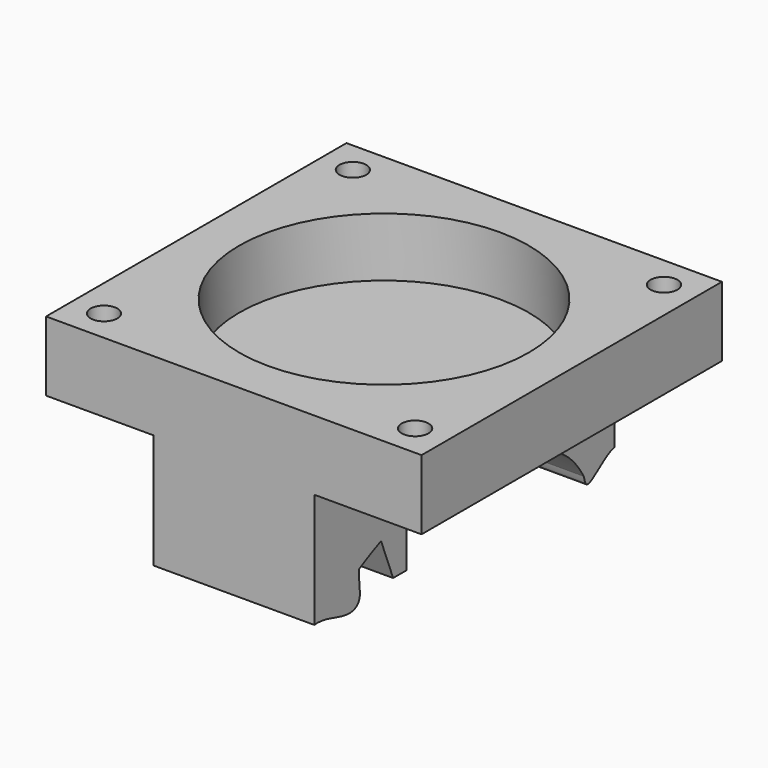
from build123d import *

# Parameters (mm, degrees)
F0_W       = 35
F0_H       = 35
F0_W_2     = 23
F0_H_2     = 23
F1_DEPTH   = 2
F3_DEPTH   = 5.5
F4_DEPTH   = 2.5
F5_DEPTH   = 1
F7_W       = 35
F7_H       = 35
F7_R       = 13.5
F8_DEPTH   = 1
F9_D       = 2.5
F9_DEPTH   = 10
F9_TIP     = 0.7510757738
F9_2_D     = 2.5
F9_2_DEPTH = 10
F9_2_TIP   = 0.7510757738
F10_W      = 7.5
F10_H      = 17.5
F11_DEPTH  = 25
F14_DEPTH  = 25


with BuildPart() as f1:
    # F0 (on Top) → F1 (new body)
    with BuildSketch(Plane.XY):
        with Locations((-9.5, 9.5)):
            Rectangle(F0_W, F0_H)
        with Locations((-9.5, 9.5)):
            Rectangle(F0_W_2, F0_H_2, mode=Mode.SUBTRACT)
        with Locations((-9.5, 9.5)):
            Rectangle(F0_W_2, F0_H_2)
        with BuildLine():
            Line((0, 5.027864045), (0, 0))
            Line((0, 0), (-5.027864045, 0))
            ThreePointArc((-5.027864045, 0), (-9.5, -1), (-13.972135955, 0))
            Line((-13.972135955, 0), (-19, 0))
            Line((-19, 0), (-19, 5.027864045))
            ThreePointArc((-19, 5.027864045), (-20, 9.5), (-19, 13.972135955))
            Line((-19, 13.972135955), (-19, 19))
            Line((-19, 19), (-13.972135955, 19))
            ThreePointArc((-13.972135955, 19), (-9.5, 20), (-5.027864045, 19))
            Line((-5.027864045, 19), (0, 19))
            Line((0, 19), (0, 13.972135955))
            ThreePointArc((0, 13.972135955), (0.746950766, 11.7912878475), (1, 9.5))
            ThreePointArc((1, 9.5), (0.746950766, 7.2087121525), (0, 5.027864045))
        make_face(mode=Mode.SUBTRACT)
        with BuildLine():
            Line((-13.972135955, 0), (-5.027864045, 0))
            ThreePointArc((-5.027864045, 0), (-2.0753787975, 2.0753787975), (0, 5.027864045))
            Line((0, 5.027864045), (0, 13.972135955))
            ThreePointArc((0, 13.972135955), (-2.0753787975, 16.9246212025), (-5.027864045, 19))
            Line((-5.027864045, 19), (-13.972135955, 19))
            ThreePointArc((-13.972135955, 19), (-16.9246212025, 16.9246212025), (-19, 13.972135955))
            Line((-19, 13.972135955), (-19, 5.027864045))
            ThreePointArc((-19, 5.027864045), (-16.9246212025, 2.0753787975), (-13.972135955, 0))
        make_face()
        with BuildLine():
            Line((-19, 19), (-19, 13.972135955))
            ThreePointArc((-19, 13.972135955), (-16.9246212025, 16.9246212025), (-13.972135955, 19))
            Line((-13.972135955, 19), (-19, 19))
        make_face()
        with BuildLine():
            ThreePointArc((-5.027864045, 19), (-2.0753787975, 16.9246212025), (0, 13.972135955))
            Line((0, 13.972135955), (0, 19))
            Line((0, 19), (-5.027864045, 19))
        make_face()
        with BuildLine():
            Line((-5.027864045, 0), (0, 0))
            Line((0, 0), (0, 5.027864045))
            ThreePointArc((0, 5.027864045), (-2.0753787975, 2.0753787975), (-5.027864045, 0))
        make_face()
        with BuildLine():
            Line((-19, 0), (-13.972135955, 0))
            ThreePointArc((-13.972135955, 0), (-16.9246212025, 2.0753787975), (-19, 5.027864045))
            Line((-19, 5.027864045), (-19, 0))
        make_face()
        with BuildLine():
            Line((0, 13.972135955), (0, 5.027864045))
            ThreePointArc((0, 5.027864045), (0.746950766, 7.2087121525), (1, 9.5))
            ThreePointArc((1, 9.5), (0.746950766, 11.7912878475), (0, 13.972135955))
        make_face()
        with BuildLine():
            ThreePointArc((-13.972135955, 0), (-9.5, -1), (-5.027864045, 0))
            Line((-5.027864045, 0), (-13.972135955, 0))
        make_face()
        with BuildLine():
            ThreePointArc((-19, 13.972135955), (-20, 9.5), (-19, 5.027864045))
            Line((-19, 5.027864045), (-19, 13.972135955))
        make_face()
        with BuildLine():
            Line((-13.972135955, 19), (-5.027864045, 19))
            ThreePointArc((-5.027864045, 19), (-9.5, 20), (-13.972135955, 19))
        make_face()
    extrude(amount=-F1_DEPTH)

    # F0 (on Top) → F4 (join)
    with BuildSketch(Plane.XY):
        with Locations((-9.5, 9.5)):
            Rectangle(F0_W_2, F0_H_2)
        with BuildLine():
            Line((0, 5.027864045), (0, 0))
            Line((0, 0), (-5.027864045, 0))
            ThreePointArc((-5.027864045, 0), (-9.5, -1), (-13.972135955, 0))
            Line((-13.972135955, 0), (-19, 0))
            Line((-19, 0), (-19, 5.027864045))
            ThreePointArc((-19, 5.027864045), (-20, 9.5), (-19, 13.972135955))
            Line((-19, 13.972135955), (-19, 19))
            Line((-19, 19), (-13.972135955, 19))
            ThreePointArc((-13.972135955, 19), (-9.5, 20), (-5.027864045, 19))
            Line((-5.027864045, 19), (0, 19))
            Line((0, 19), (0, 13.972135955))
            ThreePointArc((0, 13.972135955), (0.746950766, 11.7912878475), (1, 9.5))
            ThreePointArc((1, 9.5), (0.746950766, 7.2087121525), (0, 5.027864045))
        make_face(mode=Mode.SUBTRACT)
        with BuildLine():
            ThreePointArc((-19, 13.972135955), (-20, 9.5), (-19, 5.027864045))
            Line((-19, 5.027864045), (-19, 13.972135955))
        make_face()
        with BuildLine():
            Line((-13.972135955, 19), (-5.027864045, 19))
            ThreePointArc((-5.027864045, 19), (-9.5, 20), (-13.972135955, 19))
        make_face()
        with BuildLine():
            Line((0, 13.972135955), (0, 5.027864045))
            ThreePointArc((0, 5.027864045), (0.746950766, 7.2087121525), (1, 9.5))
            ThreePointArc((1, 9.5), (0.746950766, 11.7912878475), (0, 13.972135955))
        make_face()
        with BuildLine():
            ThreePointArc((-13.972135955, 0), (-9.5, -1), (-5.027864045, 0))
            Line((-5.027864045, 0), (-13.972135955, 0))
        make_face()
    extrude(amount=F4_DEPTH)


with BuildPart() as f3:
    # F2 (on face) → F3 (new body)
    with BuildSketch(Plane(origin=(0, 0, -2), x_dir=(1, 0, 0), z_dir=(0, 0, -1))):
        with BuildLine():
            Line((-27, -9.5), (-27, -27))
            Line((-27, -27), (8, -27))
            Line((8, -27), (8, -9.5))
            Line((8, -9.5), (4, -9.5))
            ThreePointArc((4, -9.5), (-9.5, -23), (-23, -9.5))
            Line((-23, -9.5), (-27, -9.5))
        make_face()
        with BuildLine():
            Line((-27, 8), (-27, -9.5))
            Line((-27, -9.5), (-23, -9.5))
            ThreePointArc((-23, -9.5), (-9.5, 4), (4, -9.5))
            Line((4, -9.5), (8, -9.5))
            Line((8, -9.5), (8, 8))
            Line((8, 8), (-27, 8))
        make_face()
    extrude(amount=F3_DEPTH)


with BuildPart() as f5:
    # F5 (new): a face of the model
    f5_faces = [f3.part.faces().sort_by_distance(p)[0] for p in [
        (-9.5, 26.5050252532, -7.5),
    ]]
    extrude(f5_faces, amount=F5_DEPTH)


with BuildPart() as f5b:
    # F5#2 (new): a face of the model
    f5_2_faces = [f1.part.faces().sort_by_distance(p)[0] for p in [
        (-9.5, 9.5, -2),
    ]]
    extrude(f5_2_faces, amount=F5_DEPTH)


with BuildPart() as f3_1:
    add(f3.part)

    # F7 (on face) → F8 (join)
    with BuildSketch(Plane(origin=(0, 0, -7.5), x_dir=(1, 0, 0), z_dir=(0, 0, -1))):
        with Locations((-9.5, -9.5)):
            Rectangle(F7_W, F7_H)
        with Locations((-9.5, -9.5)):
            Circle(F7_R, mode=Mode.SUBTRACT)
        with Locations((-9.5, -9.5)):
            Circle(F7_R)
    extrude(amount=F8_DEPTH)

    # F9#2
    with Locations(Plane.XY):
        with Locations((-24, -5), (-24, 24), (5, 24), (5, -5)):
            Hole(F9_2_D / 2, depth=F9_2_DEPTH)
            with Locations((0, 0, -(F9_2_DEPTH + F9_2_TIP / 2))):  # 118° drill point
                Cone(0, F9_2_D / 2, F9_2_TIP, mode=Mode.SUBTRACT)

    # F10 (on face) → F11 (join)
    with BuildSketch(Plane(origin=(0, 0, -8.5), x_dir=(1, 0, 0), z_dir=(0, 0, -1))):
        with Locations((-13.25, -0.75)):
            Rectangle(F10_W, F10_H)
        with Locations((-13.25, -18.25)):
            Rectangle(F10_W, F10_H)
        Polygon((-2, 8), (-9.5, 8), (-9.5, -9.5), (-9.5, -27), (-2, -27), (-2, -9.5), align=None)
    extrude(amount=F11_DEPTH)

    # F12 (on face) → F14 (cut)
    with BuildSketch(Plane(origin=(-17, 0, 0), x_dir=(0, -1, 0), z_dir=(-1, 0, 0))):
        with BuildLine():
            ThreePointArc((8, -20.6464289286), (10.2622326081, -23.1881038946), (12.1583798804, -26.0134239698))
            add(Edge.make_bspline(
                [(9.5055997309, -19.87504685), (10.8127451944, -21.0637318145), (11.7682585156, -23.7020451145), (12.1583798804, -26.0134239698)],
                knots=[0.8657588286, 0.8657588286, 0.8657588286, 0.8657588286, 0.9023982432, 0.9023982432, 0.9023982432, 0.9023982432], degree=3))
            add(Edge.make_bspline(
                [(8, -19.8750468523), (8.5018665766, -19.8750468523), (9.0037331533, -19.8750468523), (9.5055997299, -19.8750468523)],
                knots=[3.7172860907, 3.7172860907, 3.7172860907, 3.7172860907, 5.2228858206, 5.2228858206, 5.2228858206, 5.2228858206], degree=3))
            Line((8, -19.8750468523), (8, -20.6464289286))
        make_face()
        with BuildLine():
            Line((8, -33.5), (8, -20.6464289286))
            ThreePointArc((8, -20.6464289286), (7.5926840237, -20.2560927193), (7.1766639424, -19.8750468523))
            add(Edge.make_bspline(
                [(4.2827139093, -19.8750468523), (5.2473639204, -19.8750468523), (6.2120139314, -19.8750468523), (7.1766639424, -19.8750468523)],
                knots=[0, 0, 0, 0, 2.893950033, 2.893950033, 2.893950033, 2.893950033], degree=3))
            add(Edge.make_bspline(
                [(2.8123684214, -16.7421144443), (2.8313271516, -17.6739089609), (2.3115176613, -19.5221076361), (3.4813863955, -19.974742856), (4.2827139093, -19.8750468523)],
                knots=[0.7747233565, 0.7747233565, 0.7747233565, 0.7747233565, 0.7975926708, 0.8215331441, 0.8215331441, 0.8215331441, 0.8215331441], degree=3))
            ThreePointArc((2.8123684214, -16.7421144443), (1.5330862408, -16.0662974968), (0.2168513163, -15.4656169933))
            Line((0.2168513163, -15.4656169933), (-1.1886953891, -19.0725976635))
            Line((-1.1886953891, -19.0725976635), (-2.7616880212, -19.0725976635))
            Line((-2.7616880212, -19.0725976635), (-2.7616880212, -14.4252175155))
            ThreePointArc((-2.7616880212, -14.4252175155), (-4.6163350856, -13.9816432646), (-6.4993970616, -13.6807255947))
            add(Edge.make_bspline(
                [(-9.2018268506, -13.5017782078), (-9.2990057713, -13.9988820879), (-9.5511018083, -14.8048690203), (-6.8368571206, -16.1704874293), (-6.8719374268, -14.3568034615), (-6.4993970616, -13.6807255947)],
                knots=[0.6327799253, 0.6327799253, 0.6327799253, 0.6327799253, 0.6515188161, 0.6774841861, 0.7000997805, 0.7000997805, 0.7000997805, 0.7000997805], degree=3))
            ThreePointArc((-9.2018268506, -13.5017782078), (-10.8614735235, -13.5370997309), (-12.5151173515, -13.6824846659))
            add(Edge.make_bspline(
                [(-15.2431377999, -14.1686135165), (-15.2230914617, -14.186490334), (-14.5110157788, -14.7775282115), (-13.1041688105, -14.3832573209), (-12.5151173515, -13.6824846659)],
                knots=[0.5073436732, 0.5073436732, 0.5073436732, 0.5073436732, 0.508181821, 0.5363166804, 0.5363166804, 0.5363166804, 0.5363166804], degree=3))
            ThreePointArc((-15.2431377999, -14.1686135165), (-16.4024148058, -14.471752668), (-17.5458348497, -14.8300920667))
            add(Edge.make_bspline(
                [(-18.1226869801, -15.0340828169), (-17.8027316743, -14.9826221458), (-17.5811449306, -14.9415077326), (-17.5458348497, -14.8300920667)],
                knots=[0.4031741859, 0.4031741859, 0.4031741859, 0.4031741859, 0.4147354435, 0.4147354435, 0.4147354435, 0.4147354435], degree=3))
            ThreePointArc((-18.1226869801, -15.0340828169), (-18.1900506131, -15.0589458355), (-18.2573425562, -15.0840022345))
            add(Edge.make_bspline(
                [(-19.6143379019, -15.9263108478), (-19.0236803177, -15.8284887287), (-18.4325706363, -15.7305094799), (-18.2573425562, -15.0840022345)],
                knots=[0, 0, 0, 0, 0.3917840396, 0.3917840396, 0.3917840396, 0.3917840396], degree=3))
            add(Edge.make_bspline(
                [(-23.4159896752, -19.7753883811), (-22.9721244256, -19.0283897834), (-21.8974225661, -17.4306348464), (-20.101052847, -16.3870966389), (-19.6143379019, -15.9263108478)],
                knots=[0.1111020417, 0.1111020417, 0.1111020417, 0.1111020417, 0.4183213278, 0.795391925, 0.795391925, 0.795391925, 0.795391925], degree=3))
            add(Edge.make_bspline(
                [(-23.8874395893, -20.5935771198), (-23.6010567231, -20.6084201072), (-23.5234236473, -20.2613632826), (-23.4159896752, -19.7753883811)],
                knots=[0.3253369552, 0.3253369552, 0.3253369552, 0.3253369552, 0.341239533, 0.341239533, 0.341239533, 0.341239533], degree=3))
            add(Edge.make_bspline(
                [(-25.6971403067, -19.4565589799), (-24.9668909667, -19.9589300186), (-24.2551199556, -20.5745205502), (-23.8874395893, -20.5935771198)],
                knots=[0.3049200018, 0.3049200018, 0.3049200018, 0.3049200018, 0.3253369552, 0.3253369552, 0.3253369552, 0.3253369552], degree=3))
            ThreePointArc((-25.6971403067, -19.4565589799), (-26.3590706694, -20.0399963119), (-27, -20.6464289286))
            Line((-27, -20.6464289286), (-27, -22.1585663454))
            add(Edge.make_bspline(
                [(-27, -26.6062420868), (-26.5055885877, -27.0965498322), (-25.0286009249, -28.3702450045), (-22.9820559568, -24.2664373814), (-25.9708856134, -22.9525133649), (-27, -22.1585663454)],
                knots=[0.1717715829, 0.1717715829, 0.1717715829, 0.1717715829, 0.1873462046, 0.2199309977, 0.2499693636, 0.2499693636, 0.2499693636, 0.2499693636], degree=3))
            Line((-27, -26.6062420868), (-27, -33.5))
            Line((-27, -33.5), (-9.5, -33.5))
            Line((-9.5, -33.5), (8, -33.5))
        make_face()
        with BuildLine():
            ThreePointArc((7.1766639424, -19.8750468523), (7.5926840237, -20.2560927193), (8, -20.6464289286))
            Line((8, -20.6464289286), (8, -19.8750468523))
            add(Edge.make_bspline(
                [(7.1766639424, -19.8750468523), (7.4511092949, -19.8750468523), (7.7255546475, -19.8750468523), (8, -19.8750468523)],
                knots=[2.893950033, 2.893950033, 2.893950033, 2.893950033, 3.7172860907, 3.7172860907, 3.7172860907, 3.7172860907], degree=3))
        make_face()
        with BuildLine():
            Line((-27, -18.8217418056), (-27, -20.6464289286))
            ThreePointArc((-27, -20.6464289286), (-26.3590706694, -20.0399963119), (-25.6971403067, -19.4565589799))
            add(Edge.make_bspline(
                [(-27, -18.8217418056), (-26.610452829, -18.8767324611), (-26.1502396227, -19.1448517842), (-25.6971403067, -19.4565589799)],
                knots=[0.2922518526, 0.2922518526, 0.2922518526, 0.2922518526, 0.3049200018, 0.3049200018, 0.3049200018, 0.3049200018], degree=3))
        make_face()
        with BuildLine():
            add(Edge.make_bspline(
                [(-27, -26.6062420868), (-26.5055885877, -27.0965498322), (-25.0286009249, -28.3702450045), (-22.9820559568, -24.2664373814), (-25.9708856134, -22.9525133649), (-27, -22.1585663454)],
                knots=[0.1717715829, 0.1717715829, 0.1717715829, 0.1717715829, 0.1873462046, 0.2199309977, 0.2499693636, 0.2499693636, 0.2499693636, 0.2499693636], degree=3))
            Line((-27, -22.1585663454), (-27, -26.6062420868))
        make_face()
        with BuildLine():
            add(Edge.make_bspline(
                [(4.2827139093, -19.8750468523), (5.2473639204, -19.8750468523), (6.2120139314, -19.8750468523), (7.1766639424, -19.8750468523)],
                knots=[0, 0, 0, 0, 2.893950033, 2.893950033, 2.893950033, 2.893950033], degree=3))
            ThreePointArc((7.1766639424, -19.8750468523), (6.8538807813, -19.590992004), (6.5262601128, -19.3125304743))
            add(Edge.make_bspline(
                [(4.2827139093, -19.8750468523), (4.9334271801, -19.7940893019), (5.7180070677, -19.4947382557), (6.5262601128, -19.3125304743)],
                knots=[0.8215331441, 0.8215331441, 0.8215331441, 0.8215331441, 0.8409738639, 0.8409738639, 0.8409738639, 0.8409738639], degree=3))
        make_face()
        with BuildLine():
            ThreePointArc((6.5262601128, -19.3125304743), (6.8538807813, -19.590992004), (7.1766639424, -19.8750468523))
            add(Edge.make_bspline(
                [(7.1766639424, -19.8750468523), (7.4511092949, -19.8750468523), (7.7255546475, -19.8750468523), (8, -19.8750468523)],
                knots=[2.893950033, 2.893950033, 2.893950033, 2.893950033, 3.7172860907, 3.7172860907, 3.7172860907, 3.7172860907], degree=3))
            Line((8, -19.8750468523), (8, -19.1852972074))
            add(Edge.make_bspline(
                [(6.5262601128, -19.3125304743), (7.0170011902, -19.2019007112), (7.5164692945, -19.1344554036), (8, -19.1852972074)],
                knots=[0.8409738639, 0.8409738639, 0.8409738639, 0.8409738639, 0.8527775433, 0.8527775433, 0.8527775433, 0.8527775433], degree=3))
        make_face()
        with BuildLine():
            add(Edge.make_bspline(
                [(-18.2573425562, -15.0840022345), (-18.2547058562, -15.0742740809), (-18.2521633199, -15.0644217298), (-18.2497163658, -15.0544433129)],
                knots=[0.3917840396, 0.3917840396, 0.3917840396, 0.3917840396, 0.3976793105, 0.3976793105, 0.3976793105, 0.3976793105], degree=3))
            ThreePointArc((-18.2573425562, -15.0840022345), (-18.1900506131, -15.0589458355), (-18.1226869801, -15.0340828169))
            add(Edge.make_bspline(
                [(-18.2497163658, -15.0544433129), (-18.2058949265, -15.0473766922), (-18.1634910196, -15.0406456187), (-18.1226869801, -15.0340828169)],
                knots=[0.4016997737, 0.4016997737, 0.4016997737, 0.4016997737, 0.4031741859, 0.4031741859, 0.4031741859, 0.4031741859], degree=3))
        make_face()
        with BuildLine():
            add(Edge.make_bspline(
                [(-18.2497163658, -15.0544433129), (-18.1780472404, -14.7621842896), (-18.1883735317, -14.3617794246), (-18.23863969, -13.9514878708)],
                knots=[0.3976793105, 0.3976793105, 0.3976793105, 0.3976793105, 0.5703465901, 0.5703465901, 0.5703465901, 0.5703465901], degree=3))
            add(Edge.make_bspline(
                [(-18.2497163658, -15.0544433129), (-18.2058949265, -15.0473766922), (-18.1634910196, -15.0406456187), (-18.1226869801, -15.0340828169)],
                knots=[0.4016997737, 0.4016997737, 0.4016997737, 0.4016997737, 0.4031741859, 0.4031741859, 0.4031741859, 0.4031741859], degree=3))
            ThreePointArc((-18.1226869801, -15.0340828169), (-17.8348850055, -14.9303226168), (-17.5458348497, -14.8300920667))
            add(Edge.make_bspline(
                [(-17.5458348497, -14.8300920667), (-17.5401991962, -14.8123096069), (-17.5324447109, -14.6418665619), (-17.9116079868, -14.3107647935), (-18.23863969, -13.9514878708)],
                knots=[0.4147354435, 0.4147354435, 0.4147354435, 0.4147354435, 0.4165806741, 0.4308036025, 0.4308036025, 0.4308036025, 0.4308036025], degree=3))
        make_face()
        with BuildLine():
            ThreePointArc((-17.5458348497, -14.8300920667), (-17.8348850055, -14.9303226168), (-18.1226869801, -15.0340828169))
            add(Edge.make_bspline(
                [(-18.1226869801, -15.0340828169), (-17.8027316743, -14.9826221458), (-17.5811449306, -14.9415077326), (-17.5458348497, -14.8300920667)],
                knots=[0.4031741859, 0.4031741859, 0.4031741859, 0.4031741859, 0.4147354435, 0.4147354435, 0.4147354435, 0.4147354435], degree=3))
        make_face()
        with BuildLine():
            add(Edge.make_bspline(
                [(-18.23863969, -13.9514878708), (-18.2641252879, -13.7434647019), (-18.2998779169, -13.5329000388), (-18.3404163132, -13.3326003803)],
                knots=[0.5703465901, 0.5703465901, 0.5703465901, 0.5703465901, 0.6578911528, 0.6578911528, 0.6578911528, 0.6578911528], degree=3))
            add(Edge.make_bspline(
                [(-17.5458348497, -14.8300920667), (-17.5401991962, -14.8123096069), (-17.5324447109, -14.6418665619), (-17.9116079868, -14.3107647935), (-18.23863969, -13.9514878708)],
                knots=[0.4147354435, 0.4147354435, 0.4147354435, 0.4147354435, 0.4165806741, 0.4308036025, 0.4308036025, 0.4308036025, 0.4308036025], degree=3))
            ThreePointArc((-17.5458348497, -14.8300920667), (-16.4024148058, -14.471752668), (-15.2431377999, -14.1686135165))
            add(Edge.make_bspline(
                [(-16.0930166179, -12.2592074572), (-15.8719007213, -12.9382844563), (-15.703065724, -13.7584614246), (-15.2431377999, -14.1686135165)],
                knots=[0.4881138481, 0.4881138481, 0.4881138481, 0.4881138481, 0.5073436732, 0.5073436732, 0.5073436732, 0.5073436732], degree=3))
            add(Edge.make_bspline(
                [(-16.0967430478, -12.24779185), (-16.0954992187, -12.2515925467), (-16.0942570956, -12.2553977815), (-16.0930166179, -12.2592074572)],
                knots=[0.4880059672, 0.4880059672, 0.4880059672, 0.4880059672, 0.4881138481, 0.4881138481, 0.4881138481, 0.4881138481], degree=3))
            add(Edge.make_bspline(
                [(-18.3404163132, -13.3326003803), (-17.2526634188, -12.7769450369), (-16.1622180551, -12.2200414159), (-16.0967430478, -12.24779185)],
                knots=[0, 0, 0, 0, 0.9350904711, 0.9350904711, 0.9350904711, 0.9350904711], degree=3))
        make_face()
        with BuildLine():
            add(Edge.make_bspline(
                [(-18.3404163132, -13.3326003803), (-18.4681622578, -12.7014094243), (-18.6434321703, -12.1721527486), (-18.6947030438, -12.1455790189)],
                knots=[0.6578911528, 0.6578911528, 0.6578911528, 0.6578911528, 0.9337644949, 0.9337644949, 0.9337644949, 0.9337644949], degree=3))
            add(Edge.make_bspline(
                [(-18.3404163132, -13.3326003803), (-17.2526634188, -12.7769450369), (-16.1622180551, -12.2200414159), (-16.0967430478, -12.24779185)],
                knots=[0, 0, 0, 0, 0.9350904711, 0.9350904711, 0.9350904711, 0.9350904711], degree=3))
            add(Edge.make_bspline(
                [(-18.6947030438, -12.1455790189), (-18.2868799319, -11.4854053666), (-16.7427265833, -10.68299329), (-16.2513567713, -11.7753476578), (-16.0967430478, -12.24779185)],
                knots=[0.4515959411, 0.4515959411, 0.4515959411, 0.4515959411, 0.4745958795, 0.4880059672, 0.4880059672, 0.4880059672, 0.4880059672], degree=3))
        make_face()
        with BuildLine():
            ThreePointArc((-12.5151173515, -13.6824846659), (-10.8614735235, -13.5370997309), (-9.2018268506, -13.5017782078))
            add(Edge.make_bspline(
                [(-9.1493576349, -11.6850000157), (-9.0727226024, -12.2053870207), (-9.0907871476, -12.8961106994), (-9.1831488747, -13.4062338836), (-9.2018268506, -13.5017782078)],
                knots=[0.6146656397, 0.6146656397, 0.6146656397, 0.6146656397, 0.6291782743, 0.6327799253, 0.6327799253, 0.6327799253, 0.6327799253], degree=3))
            add(Edge.make_bspline(
                [(-12.3073167066, -11.5099274874), (-11.2556032541, -11.5683159988), (-10.2010710874, -11.6266115042), (-9.1493576349, -11.6850000157)],
                knots=[0, 0, 0, 0, 3.1628082283, 3.1628082283, 3.1628082283, 3.1628082283], degree=3))
            add(Edge.make_bspline(
                [(-12.5151173515, -13.6824846659), (-12.4482546026, -13.6029405356), (-12.0136270301, -12.9635019395), (-12.2866289866, -12.1369062713), (-12.3073167066, -11.5099274874)],
                knots=[0.5363166804, 0.5363166804, 0.5363166804, 0.5363166804, 0.5395102452, 0.5607318503, 0.5607318503, 0.5607318503, 0.5607318503], degree=3))
        make_face()
        with BuildLine():
            add(Edge.make_bspline(
                [(-12.3073167066, -11.5099274874), (-11.2556032541, -11.5683159988), (-10.2010710874, -11.6266115042), (-9.1493576349, -11.6850000157)],
                knots=[0, 0, 0, 0, 3.1628082283, 3.1628082283, 3.1628082283, 3.1628082283], degree=3))
            add(Edge.make_bspline(
                [(-12.3073167066, -11.5099274874), (-12.3153570658, -11.2662498573), (-12.2065681432, -10.2529703979), (-9.8307339349, -9.5424352975), (-9.2421623139, -11.0548136972), (-9.1493576349, -11.6850000157)],
                knots=[0.5607318503, 0.5607318503, 0.5607318503, 0.5607318503, 0.5689797058, 0.5970909045, 0.6146656397, 0.6146656397, 0.6146656397, 0.6146656397], degree=3))
        make_face()
    extrude(amount=-F14_DEPTH, mode=Mode.SUBTRACT)


with BuildPart() as f1_1:
    add(f1.part)

    # F9
    with Locations(Plane.XY):
        with Locations((-24, -5), (-24, 24), (5, 24), (5, -5)):
            Hole(F9_D / 2, depth=F9_DEPTH)
            with Locations((0, 0, -(F9_DEPTH + F9_TIP / 2))):  # 118° drill point
                Cone(0, F9_D / 2, F9_TIP, mode=Mode.SUBTRACT)


solid = f3_1.part
